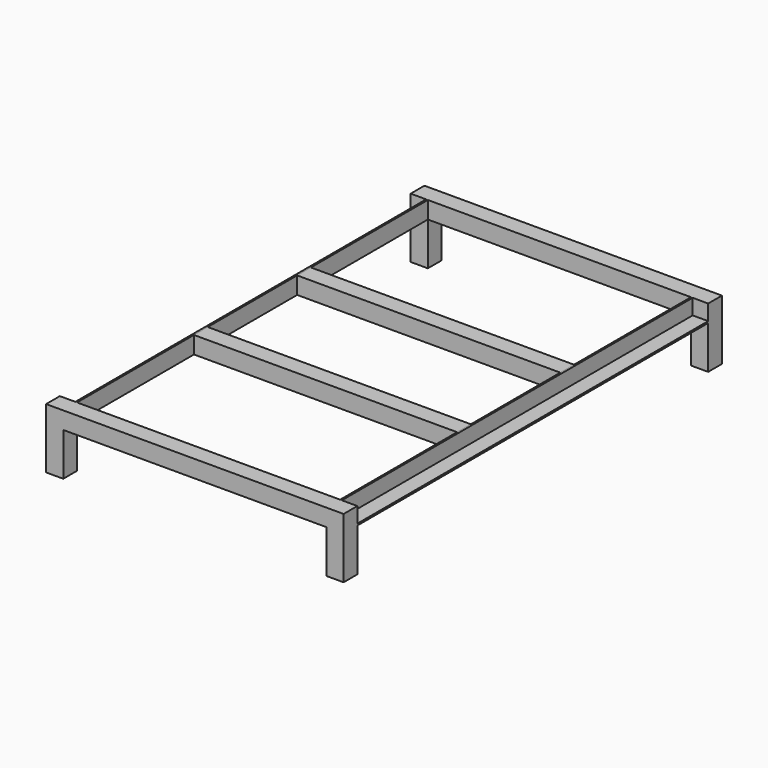
from build123d import *

# Parameters (mm, degrees)
F1_DEPTH = 510
F3_DEPTH = 40
F4_W     = 612
F4_H     = 40
F5_DEPTH = 40


# Not quite as in the source:
# - a pattern or mirror of a feature is missing from the dataset's text; its kind, count and spacing are read off the source's solid


with BuildPart() as f1:
    # F0 (on Front) → F1 (new body, symmetric)
    with BuildSketch(Plane.XZ):
        Polygon((310, -36), (310, 0), (306, 0), (306, -40), (346, -40), (346, -36), align=None)
    extrude(amount=F1_DEPTH, both=True)


with BuildPart() as f1_copies_1:
    # F1_copies: instance of F1
    add(f1.part.mirror(Plane(origin=(0, 0, 0), x_dir=(0, 0, -1), z_dir=(-1, 0, 0))))


with BuildPart() as f3:
    # F2 (on face) → F3 (new body)
    with BuildSketch(Plane.XZ.offset(510)):
        Polygon((-306, -40), (306, -40), (306, -140), (346, -140), (346, 0), (-346, 0), (-346, -140), (-306, -140), align=None)
    extrude(amount=F3_DEPTH)


with BuildPart() as f3_copies_1:
    # F3_copies: instance of F3
    add(f3.part.mirror(Plane.ZX))


with BuildPart() as f5:
    # F4 (on face) → F5 (new body)
    with BuildSketch(Plane.XY):
        with Locations((0, 150)):
            Rectangle(F4_W, F4_H)
    extrude(amount=-F5_DEPTH)


with BuildPart() as f5_copies_1:
    # F5_copies: instance of F5
    add(f5.part.mirror(Plane(origin=(0, 0, 0), x_dir=(0, 0, -1), z_dir=(0, -1, 0))))


solid = Compound([f1.part, f1_copies_1.part, f3.part, f3_copies_1.part, f5.part, f5_copies_1.part])
